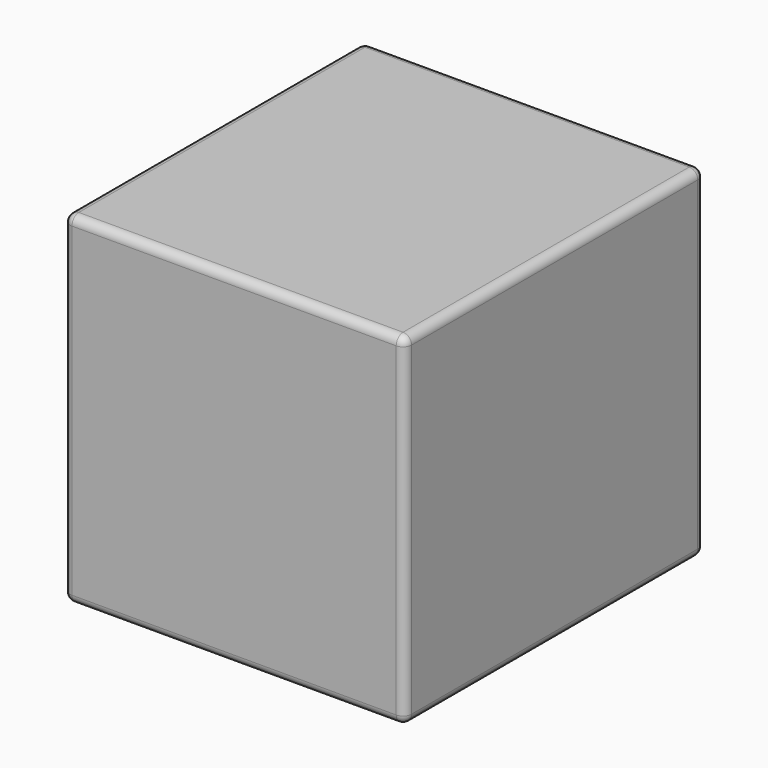
from build123d import *

# Parameters (mm, degrees)
F0_W      = 200.3522217274
F0_H      = 200.7694281638
F1_DEPTH  = 220
F2_W      = 106.5517105162
F2_H      = 12.7497781068
F3_DEPTH  = 15
F4_R      = 5
F5_R      = 5
F6_R      = 5
F8_R      = 5
F9_R      = 5
F12_DEPTH = 6.66
F14_R     = 8.8266857578
F14_R_2   = 8.8654347792
F14_R_3   = 9.3130675206
F14_R_4   = 9.3531300043
F15_DEPTH = 7
F7_R      = 11.1504231151
F18_DEPTH = 2


# Not quite as in the source:
# - the program builds the solid bodies; features that only make, move or delete a surface that nothing else refers to are left out


with BuildPart() as f1:
    # F0 (on Front) → F1 (new body)
    with BuildSketch(Plane.XZ):
        with Locations((35.5218797922, -56.1928581446)):
            Rectangle(F0_W, F0_H)
    extrude(amount=F1_DEPTH)

    # F2 (on face) → F3 (join)
    with BuildSketch(Plane.XZ.offset(220)):
        with Locations((33.8400062174, 20.9869192913)):
            Rectangle(F2_W, F2_H)
    extrude(amount=-F3_DEPTH)

    # F4
    f4_edges = [f1.edges().sort_by_distance(p)[0] for p in [
        (35.52188, -220, 44.191856),
    ]]
    fillet(f4_edges, radius=F4_R)

    # F5
    f5_edges = [f1.edges().sort_by_distance(p)[0] for p in [
        (135.697991, -218.535534, 42.72739),
    ]]
    fillet(f5_edges, radius=F5_R)

    # F6
    f6_edges = [f1.edges().sort_by_distance(p)[0] for p in [
        (-64.654231, -218.535534, 42.72739),
    ]]
    fillet(f6_edges, radius=F6_R)

    # F8
    f8_edges = [f1.edges().sort_by_distance(p)[0] for p in [
        (135.697991, -107.5, -156.577572),
        (35.52188, -220, -156.577572),
        (-64.654231, -107.5, -156.577572),
    ]]
    fillet(f8_edges, radius=F8_R)

    # F9
    f9_edges = [f1.edges().sort_by_distance(p)[0] for p in [
        (35.52188, 0, -156.577572),
    ]]
    fillet(f9_edges, radius=F9_R)

    # F2 (on face) → F12 (join)
    with BuildSketch(Plane.XZ.offset(220)):
        with Locations((33.8400062174, 20.9869192913)):
            Rectangle(F2_W, F2_H)
    extrude(amount=-F12_DEPTH)

    # F14 (on face) → F15 (join)
    with BuildSketch(Plane(origin=(0, 0, -156.5775722265), x_dir=(1, 0, 0), z_dir=(0, 0, -1))):
        with Locations((105.7562977076, 196.8253701925)):
            Circle(F14_R)
        with Locations((105.7562977076, 19.2491486669)):
            Circle(F14_R_2)
        with Locations((-43.5114949942, 20.4882938415)):
            Circle(F14_R_3)
        with Locations((-43.5114949942, 196.0519701242)):
            Circle(F14_R_4)
    extrude(amount=F15_DEPTH)

    # F7 (on face) → F18 (join)
    with BuildSketch(Plane(origin=(-64.6542310715, 0, 0), x_dir=(0, -1, 0), z_dir=(-1, 0, 0))):
        with Locations((199.0269720554, 21.7568427324)):
            Circle(F7_R)
    extrude(amount=F18_DEPTH)


solid = f1.part
